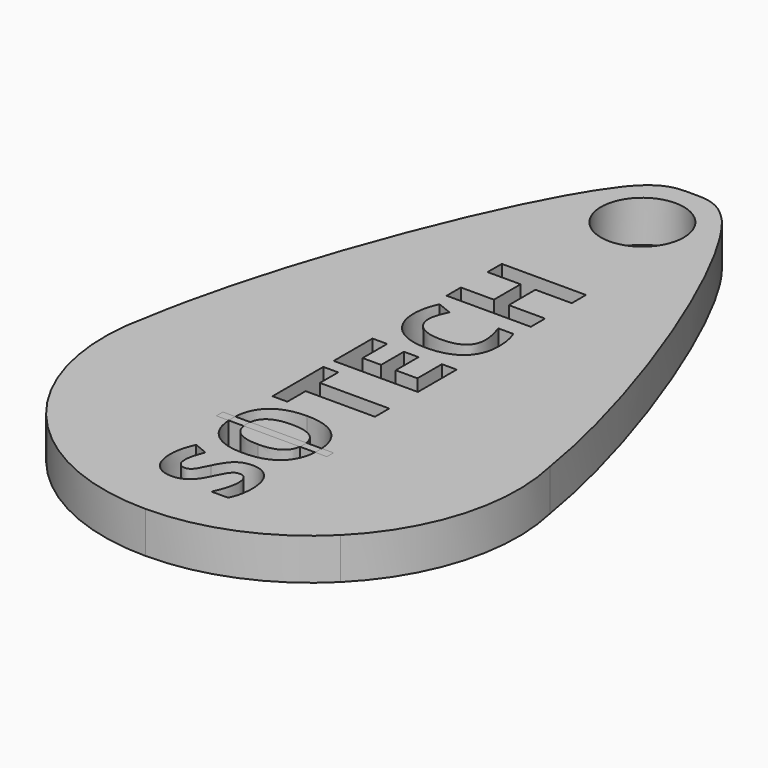
from build123d import *

# Parameters (mm, degrees)
F0_R         = 2.5
F1_DEPTH     = 2.5
F2_TEXT_SIZE = 7.1194530966
F3_DEPTH     = 25
F5_DEPTH     = 2.5


# Not quite as in the source:
# - Text() gives the source's letters only with a copy of the font that has no kerning and outlines rounded to 1/6400 em; it was checked with that copy


with BuildPart() as f1:
    # F0 (on Top) → F1 (new body)
    with BuildSketch(Plane.XY):
        with BuildLine():
            add(Edge.make_bspline(
                [(12.5, 0), (12.4512299479, 0.8609280977), (12.3413241233, 1.8056638138), (12.1797513897, 2.8113441776)],
                knots=[0.7325943199, 0.7325943199, 0.7325943199, 0.7325943199, 0.7539858989, 0.7539858989, 0.7539858989, 0.7539858989], degree=3))
            ThreePointArc((12.5, 0), (12.419679794, 1.414762812), (12.1797513897, 2.8113441776))
        make_face()
        with BuildLine():
            ThreePointArc((8.8388347648, -8.8388347648), (11.5484941564, -4.7835429046), (12.5, 0))
            add(Edge.make_bspline(
                [(12.5, 0), (12.4512299479, 0.8609280977), (12.3413241233, 1.8056638138), (12.1797513897, 2.8113441776)],
                knots=[0.7325943199, 0.7325943199, 0.7325943199, 0.7325943199, 0.7539858989, 0.7539858989, 0.7539858989, 0.7539858989], degree=3))
            ThreePointArc((12.1797513897, 2.8113441776), (0, 12.5), (-12.1797513897, 2.8113441776))
            add(Edge.make_bspline(
                [(-12.1797513897, 2.8113441776), (-12.3413241233, 1.8056638138), (-12.4512299479, 0.8609280977), (-12.5, 0)],
                knots=[0.2460141011, 0.2460141011, 0.2460141011, 0.2460141011, 0.2674056801, 0.2674056801, 0.2674056801, 0.2674056801], degree=3))
            ThreePointArc((-12.5, 0), (-11.5484941564, -4.7835429046), (-8.8388347648, -8.8388347648))
            add(Edge.make_bspline(
                [(-8.8388347648, -8.8388347648), (-6.45434185, -10.7937073455), (-3.2271709002, -12.5000000131), (4.96e-08, -12.5)],
                knots=[0.3837028401, 0.3837028401, 0.3837028401, 0.3837028401, 0.5, 0.5, 0.5, 0.5], degree=3))
            add(Edge.make_bspline(
                [(4.96e-08, -12.5), (3.2271709498, -12.4999999869), (6.4543418624, -10.793707339), (8.838834771, -8.8388347616)],
                knots=[0.5, 0.5, 0.5, 0.5, 0.6162971599, 0.6162971599, 0.6162971599, 0.6162971599], degree=3))
        make_face()
        with BuildLine():
            ThreePointArc((-12.1797513897, 2.8113441776), (0, 12.5), (12.1797513897, 2.8113441776))
            add(Edge.make_bspline(
                [(12.1797513897, 2.8113441776), (10.8633332676, 11.0051515495), (6.1171527077, 23.2445979449), (3.0624504486, 27.16423133)],
                knots=[0.7539858989, 0.7539858989, 0.7539858989, 0.7539858989, 0.9282743551, 0.9282743551, 0.9282743551, 0.9282743551], degree=3))
            ThreePointArc((3.0624504486, 27.16423133), (3.5739816159, 26.1354097978), (3.75, 25))
            ThreePointArc((3.75, 25), (-1.1354097978, 21.4260183841), (-3.0624504486, 27.16423133))
            add(Edge.make_bspline(
                [(-3.0624504486, 27.16423133), (-6.1171527077, 23.2445979449), (-10.8633332676, 11.0051515495), (-12.1797513897, 2.8113441776)],
                knots=[0.0717256449, 0.0717256449, 0.0717256449, 0.0717256449, 0.2460141011, 0.2460141011, 0.2460141011, 0.2460141011], degree=3))
        make_face()
        with BuildLine():
            ThreePointArc((7.44e-08, -12.5), (4.7835429389, -11.5484941421), (8.8388347648, -8.8388347648))
            add(Edge.make_bspline(
                [(4.96e-08, -12.5), (3.2271709498, -12.4999999869), (6.4543418624, -10.793707339), (8.838834771, -8.8388347616)],
                knots=[0.5, 0.5, 0.5, 0.5, 0.6162971599, 0.6162971599, 0.6162971599, 0.6162971599], degree=3))
        make_face()
        with BuildLine():
            add(Edge.make_bspline(
                [(-12.1797513897, 2.8113441776), (-12.3413241233, 1.8056638138), (-12.4512299479, 0.8609280977), (-12.5, 0)],
                knots=[0.2460141011, 0.2460141011, 0.2460141011, 0.2460141011, 0.2674056801, 0.2674056801, 0.2674056801, 0.2674056801], degree=3))
            ThreePointArc((-12.1797513897, 2.8113441776), (-12.419679794, 1.414762812), (-12.5, 0))
        make_face()
        with BuildLine():
            add(Edge.make_bspline(
                [(3.0624504486, 27.16423133), (2.9217624168, 27.3447548179), (2.7846623068, 27.507630525), (2.6516504294, 27.6516504294)],
                knots=[0.9282743551, 0.9282743551, 0.9282743551, 0.9282743551, 0.9363014221, 0.9363014221, 0.9363014221, 0.9363014221], degree=3))
            ThreePointArc((3.0624504486, 27.16423133), (2.867425946, 27.4166854252), (2.6516504294, 27.6516504294))
        make_face()
        with BuildLine():
            ThreePointArc((3.75, 25), (3.5739816159, 26.1354097978), (3.0624504486, 27.16423133))
            add(Edge.make_bspline(
                [(3.0624504486, 27.16423133), (2.9217624168, 27.3447548179), (2.7846623068, 27.507630525), (2.6516504294, 27.6516504294)],
                knots=[0.9282743551, 0.9282743551, 0.9282743551, 0.9282743551, 0.9363014221, 0.9363014221, 0.9363014221, 0.9363014221], degree=3))
            ThreePointArc((2.6516504294, 27.6516504294), (1.4350628714, 28.4645482469), (0, 28.75))
            ThreePointArc((0, 28.75), (-1.4350628714, 28.4645482469), (-2.6516504294, 27.6516504294))
            add(Edge.make_bspline(
                [(-2.6516504294, 27.6516504294), (-2.7846623068, 27.507630525), (-2.9217624168, 27.3447548179), (-3.0624504486, 27.16423133)],
                knots=[0.0636985779, 0.0636985779, 0.0636985779, 0.0636985779, 0.0717256449, 0.0717256449, 0.0717256449, 0.0717256449], degree=3))
            ThreePointArc((-3.0624504486, 27.16423133), (-1.1354097978, 21.4260183841), (3.75, 25))
        make_face()
        with Locations((0, 25)):
            Circle(F0_R, mode=Mode.SUBTRACT)
        with BuildLine():
            ThreePointArc((-8.8388347648, -8.8388347648), (-4.7835428702, -11.5484941706), (7.44e-08, -12.5))
            add(Edge.make_bspline(
                [(-8.8388347648, -8.8388347648), (-6.45434185, -10.7937073455), (-3.2271709002, -12.5000000131), (4.96e-08, -12.5)],
                knots=[0.3837028401, 0.3837028401, 0.3837028401, 0.3837028401, 0.5, 0.5, 0.5, 0.5], degree=3))
        make_face()
        with BuildLine():
            ThreePointArc((-2.6516504294, 27.6516504294), (-2.867425946, 27.4166854252), (-3.0624504486, 27.16423133))
            add(Edge.make_bspline(
                [(-2.6516504294, 27.6516504294), (-2.7846623068, 27.507630525), (-2.9217624168, 27.3447548179), (-3.0624504486, 27.16423133)],
                knots=[0.0636985779, 0.0636985779, 0.0636985779, 0.0636985779, 0.0717256449, 0.0717256449, 0.0717256449, 0.0717256449], degree=3))
        make_face()
        with BuildLine():
            ThreePointArc((0, 28.75), (1.4350628714, 28.4645482469), (2.6516504294, 27.6516504294))
            add(Edge.make_bspline(
                [(2.6516504294, 27.6516504294), (1.5961382021, 28.794516564), (0.7980691011, 28.75), (0, 28.75)],
                knots=[0.9363014221, 0.9363014221, 0.9363014221, 0.9363014221, 1, 1, 1, 1], degree=3))
        make_face()
        with BuildLine():
            add(Edge.make_bspline(
                [(0, 28.75), (-0.7980691011, 28.75), (-1.5961382021, 28.794516564), (-2.6516504294, 27.6516504294)],
                knots=[0, 0, 0, 0, 0.0636985779, 0.0636985779, 0.0636985779, 0.0636985779], degree=3))
            ThreePointArc((-2.6516504294, 27.6516504294), (-1.4350628714, 28.4645482469), (0, 28.75))
        make_face()
    extrude(amount=F1_DEPTH)

    # F2 (on face) → F3 (cut)
    with BuildSketch(Plane.XY.offset(2.5)):
        with Locations(Location((2.5630031148, -9.5), (0, 0, 90))):
            Text('SOTECH', F2_TEXT_SIZE, font='Open Sans', font_style=FontStyle.BOLD, text_align=(TextAlign.LEFT, TextAlign.BOTTOM))
    extrude(amount=-F3_DEPTH, mode=Mode.SUBTRACT)

    # F4 (on face) → F5 (join, through all)
    with BuildSketch(Plane.XY.offset(2.5)):
        with BuildLine():
            Line((3.337262664, -2.9887443874), (3.337262664, -2.4887443874))
            Line((3.337262664, -2.4887443874), (2.6244537019, -2.4887443874))
            add(Edge.make_bspline(
                [(2.6253503836, -2.9887443874), (2.6330852312, -2.8701749355), (2.6330852312, -2.6136297274), (2.6244537019, -2.4887443874)],
                knots=[5.8931915297, 5.8931915297, 5.8931915297, 6, 6.1128297666, 6.1128297666, 6.1128297666], degree=2))
            Line((2.6253503836, -2.9887443874), (3.337262664, -2.9887443874))
        make_face()
        with BuildLine():
            add(Edge.make_bspline(
                [(-2.5916184455, -2.4887443874), (-2.5997127948, -2.6104412522), (-2.5997127948, -2.8670053392), (-2.5916904533, -2.9887443874)],
                knots=[1.8904676922, 1.8904676922, 1.8904676922, 2, 2.1094962959, 2.1094962959, 2.1094962959], degree=2))
            Line((-2.5916184455, -2.4887443874), (-3.337262664, -2.4887443874))
            Line((-3.337262664, -2.4887443874), (-3.337262664, -2.9887443874))
            Line((-3.337262664, -2.9887443874), (-2.5916904533, -2.9887443874))
        make_face()
        with BuildLine():
            add(Edge.make_bspline(
                [(2.6253503836, -2.9887443874), (2.6330852312, -2.8701749355), (2.6330852312, -2.6136297274), (2.6244537019, -2.4887443874)],
                knots=[5.8931915297, 5.8931915297, 5.8931915297, 6, 6.1128297666, 6.1128297666, 6.1128297666], degree=2))
            Line((2.6244537019, -2.4887443874), (-2.5916184455, -2.4887443874))
            add(Edge.make_bspline(
                [(-2.5916184455, -2.4887443874), (-2.5997127948, -2.6104412522), (-2.5997127948, -2.8670053392), (-2.5916904533, -2.9887443874)],
                knots=[1.8904676922, 1.8904676922, 1.8904676922, 2, 2.1094962959, 2.1094962959, 2.1094962959], degree=2))
            Line((-2.5916904533, -2.9887443874), (2.6253503836, -2.9887443874))
        make_face()
    extrude(amount=-F5_DEPTH)


solid = f1.part
